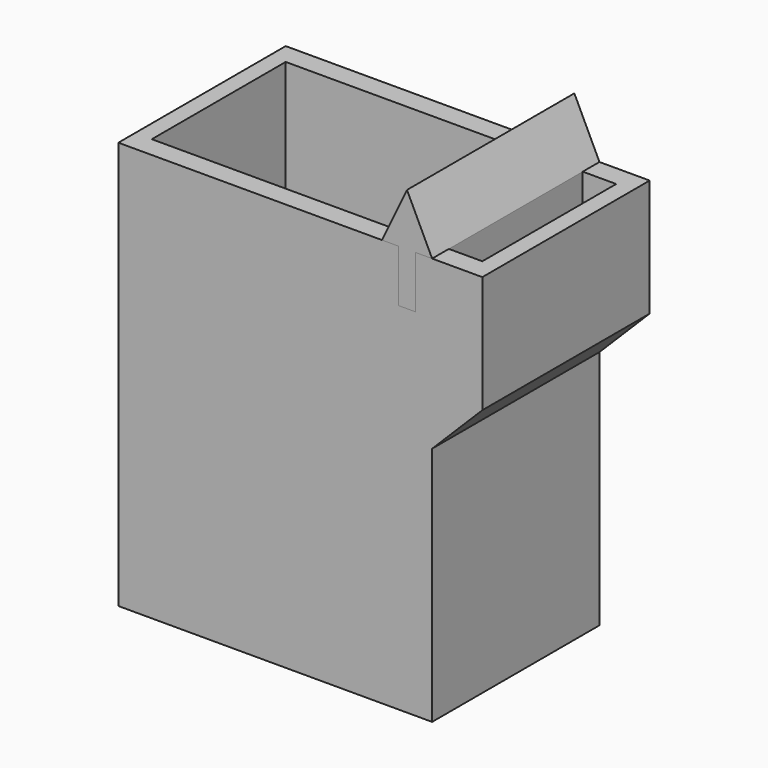
from build123d import *

# Parameters (mm, degrees)
F0_W     = 1.6
F0_H     = 37.4
F1_DEPTH = 20
F2_DEPTH = 2
F3_START = 18
F3_DEPTH = 2
F0_H_2   = 5
F4_DEPTH = 20


with BuildPart() as f1:
    # F0 (on Front) → F1 (new body)
    with BuildSketch(Plane.XZ):
        with Locations((-11.9564137042, 20.3)):
            Rectangle(F0_W, F0_H)
        Polygon((-11.1564137042, 1.6), (-12.7564137042, 1.6), (-12.7564137042, 0), (17.2435862958, 0), (17.2435862958, 1.6), (15.6435862958, 1.6), (14.0435862958, 1.6), align=None)
        Polygon((15.6435862958, 24.6), (15.6435862958, 1.6), (17.2435862958, 1.6), (17.2435862958, 23), align=None)
        Polygon((17.2435862958, 26.2), (15.6435862958, 24.6), (17.2435862958, 23), align=None)
        Polygon((17.2435862958, 26.2), (17.2435862958, 23), (22.0435862958, 27.8), (22.0435862958, 39), (20.4435862958, 39), (20.4435862958, 29.4), align=None)
    extrude(amount=F1_DEPTH)



with BuildPart() as f1b:
    # F0 (on Front) → F1, piece 2 (new body)
    with BuildSketch(Plane.XZ):
        Polygon((14.0435862958, 39), (12.4435862958, 39), (12.4435862958, 27.8), (13.2435862958, 27), (17.2435862958, 31), (17.2435862958, 39), (15.6435862958, 39), (15.6435862958, 34), (14.0435862958, 34), align=None)
    extrude(amount=F1_DEPTH)


with BuildPart() as f1_1:
    add(f1.part)

    add(f1b.part)  # F2 merges F1b
    # F0 (on Front) → F2 (join)
    with BuildSketch(Plane.XZ):
        Polygon((-11.1564137042, 39), (-11.1564137042, 1.6), (14.0435862958, 1.6), (15.6435862958, 1.6), (15.6435862958, 24.6), (13.2435862958, 27), (12.4435862958, 27.8), (12.4435862958, 39), align=None)
        Polygon((15.6435862958, 24.6), (15.6435862958, 1.6), (17.2435862958, 1.6), (17.2435862958, 23), align=None)
        Polygon((14.0435862958, 39), (12.4435862958, 39), (12.4435862958, 27.8), (13.2435862958, 27), (17.2435862958, 31), (17.2435862958, 39), (15.6435862958, 39), (15.6435862958, 34), (14.0435862958, 34), align=None)
        Polygon((13.2435862958, 27), (15.6435862958, 24.6), (17.2435862958, 26.2), (17.2435862958, 31), align=None)
        Polygon((17.2435862958, 31), (17.2435862958, 26.2), (20.4435862958, 29.4), (20.4435862958, 39), (17.2435862958, 39), align=None)
    extrude(amount=F2_DEPTH)

    # F0 (on Front) → F3 (join)
    with BuildSketch(Plane.XZ.offset(F3_START)):
        Polygon((13.2435862958, 27), (15.6435862958, 24.6), (17.2435862958, 26.2), (17.2435862958, 31), align=None)
        Polygon((17.2435862958, 26.2), (17.2435862958, 23), (22.0435862958, 27.8), (22.0435862958, 39), (20.4435862958, 39), (20.4435862958, 29.4), align=None)
        Polygon((17.2435862958, 31), (17.2435862958, 26.2), (20.4435862958, 29.4), (20.4435862958, 39), (17.2435862958, 39), align=None)
        Polygon((17.2435862958, 26.2), (15.6435862958, 24.6), (17.2435862958, 23), align=None)
        Polygon((15.6435862958, 24.6), (15.6435862958, 1.6), (17.2435862958, 1.6), (17.2435862958, 23), align=None)
        Polygon((-11.1564137042, 39), (-11.1564137042, 1.6), (14.0435862958, 1.6), (15.6435862958, 1.6), (15.6435862958, 24.6), (13.2435862958, 27), (12.4435862958, 27.8), (12.4435862958, 39), align=None)
        Polygon((-11.1564137042, 1.6), (-12.7564137042, 1.6), (-12.7564137042, 0), (17.2435862958, 0), (17.2435862958, 1.6), (15.6435862958, 1.6), (14.0435862958, 1.6), align=None)
        with Locations((-11.9564137042, 20.3)):
            Rectangle(F0_W, F0_H)
        Polygon((14.0435862958, 39), (12.4435862958, 39), (12.4435862958, 27.8), (13.2435862958, 27), (17.2435862958, 31), (17.2435862958, 39), (15.6435862958, 39), (15.6435862958, 34), (14.0435862958, 34), align=None)
    extrude(amount=F3_DEPTH)


with BuildPart() as f4:
    # F0 (on Front) → F4 (new body)
    with BuildSketch(Plane.XZ):
        Polygon((14.8435862958, 44), (12.4435862958, 39), (14.0435862958, 39), (15.6435862958, 39), (17.2435862958, 39), align=None)
        with Locations((14.8435862958, 36.5)):
            Rectangle(F0_W, F0_H_2)
    extrude(amount=F4_DEPTH)


solid = Compound([f1_1.part, f4.part])
